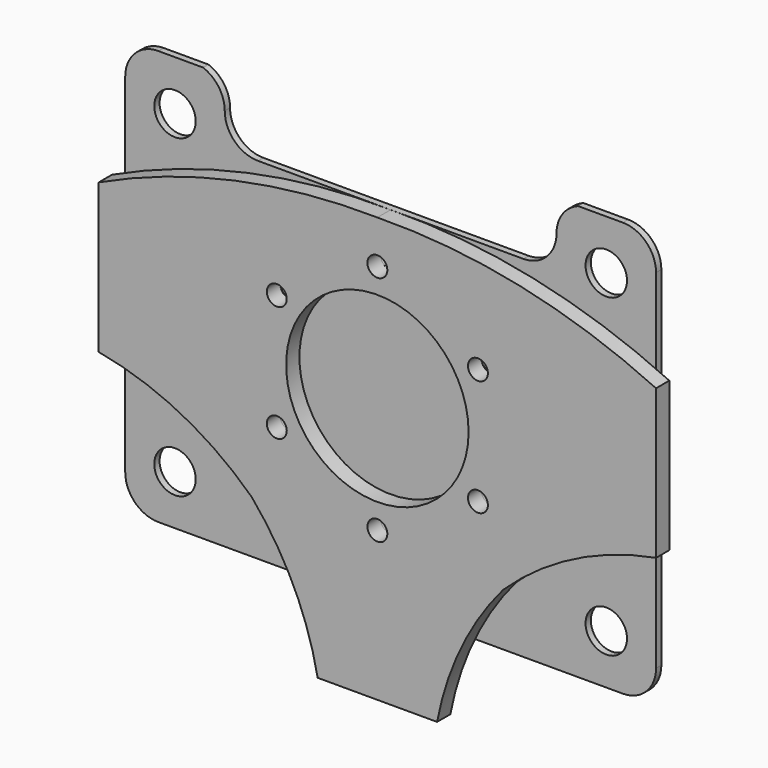
from build123d import *

# Parameters (mm, degrees)
F0_R     = 3
F1_DEPTH = 5
F2_R     = 6.25
F2_R_2   = 3
F3_DEPTH = 2


# Not quite as in the source:
# - a feature names something its author has since deleted; it is built from what else it names


with BuildPart() as f1:
    # F0 (on Front) → F1 (new body)
    with BuildSketch(Plane.XZ):
        with BuildLine():
            ThreePointArc((18, -80), (25.2450835608, -57.9435000854), (37.8911830779, -38.474124356))
            ThreePointArc((37.8911830779, -38.474124356), (59.2223421632, -23.3521866114), (84, -15))
            Line((84, -15), (84, 30))
            ThreePointArc((84, 30), (43.0306603199, 43.8097481595), (0, 48))
            ThreePointArc((0, 48), (-43.0306603199, 43.8097481595), (-84, 30))
            Line((-84, 30), (-84, -15))
            ThreePointArc((-84, -15), (-59.2223421632, -23.3521866114), (-37.8911830779, -38.474124356))
            ThreePointArc((-37.8911830779, -38.474124356), (-25.2450835608, -57.9435000854), (-18, -80))
            Line((-18, -80), (0, -80))
            Line((0, -80), (18, -80))
        make_face()
        with Locations((-30.3108891325, -17.5)):
            Circle(F0_R, mode=Mode.SUBTRACT)
        with Locations((0, -35)):
            Circle(F0_R, mode=Mode.SUBTRACT)
        with Locations((30.3108891325, -17.5)):
            Circle(F0_R, mode=Mode.SUBTRACT)
        with Locations((-30.3108891325, 17.5)):
            Circle(F0_R, mode=Mode.SUBTRACT)
        with BuildLine():
            ThreePointArc((19.2964358267, -19.5933040702), (-25.3663358138, 10.6206877076), (27.5, 0))
            ThreePointArc((27.5, 0), (25.3663358138, -10.6206877076), (19.2964358267, -19.5933040702))
        make_face(mode=Mode.SUBTRACT)
        with Locations((30.3108891325, 17.5)):
            Circle(F0_R, mode=Mode.SUBTRACT)
        with Locations((0, 35)):
            Circle(F0_R, mode=Mode.SUBTRACT)
    extrude(amount=F1_DEPTH)


with BuildPart() as f3:
    # F2 (on Front) → F3 (new body)
    with BuildSketch(Plane.XZ):
        with BuildLine():
            ThreePointArc((-40, 48), (-47.0710678119, 50.9289321881), (-50, 58))
            ThreePointArc((-50, 58), (-51.7877055527, 63.7059810647), (-56.5116439822, 67.3718393228))
            Line((-56.5116439822, 67.3718393228), (-70, 67.3718393228))
            ThreePointArc((-70, 67.3718393228), (-77.0710678119, 64.4429071347), (-80, 57.3718393228))
            Line((-80, 57.3718393228), (-80, -47.6281606772))
            ThreePointArc((-80, -47.6281606772), (-77.0710678119, -54.699228489), (-70, -57.6281606772))
            Line((-70, -57.6281606772), (0, -57.6281606772))
            Line((0, -57.6281606772), (70, -57.6281606772))
            ThreePointArc((70, -57.6281606772), (77.0710678119, -54.699228489), (80, -47.6281606772))
            Line((80, -47.6281606772), (80, 57.3718393228))
            ThreePointArc((80, 57.3718393228), (77.0710678119, 64.4429071347), (70, 67.3718393228))
            Line((70, 67.3718393228), (56.5116439822, 67.3718393228))
            ThreePointArc((56.5116439822, 67.3718393228), (51.7877055527, 63.7059810647), (50, 58))
            ThreePointArc((50, 58), (47.0710678119, 50.9289321881), (40, 48))
            Line((40, 48), (0, 48))
            Line((0, 48), (-40, 48))
        make_face()
        with Locations((-65, -42.6281606772)):
            Circle(F2_R, mode=Mode.SUBTRACT)
        with Locations((-30.3108891325, -17.6374954636)):
            Circle(F2_R_2, mode=Mode.SUBTRACT)
        with Locations((0, -35)):
            Circle(F2_R_2, mode=Mode.SUBTRACT)
        with Locations((65, -42.6281606772)):
            Circle(F2_R, mode=Mode.SUBTRACT)
        with Locations((30.3108891325, -17.6374954636)):
            Circle(F2_R_2, mode=Mode.SUBTRACT)
        with Locations((-30.3108891325, 17.6374954636)):
            Circle(F2_R_2, mode=Mode.SUBTRACT)
        with Locations((-65, 52.3718393228)):
            Circle(F2_R, mode=Mode.SUBTRACT)
        with Locations((30.3108891325, 17.6374954636)):
            Circle(F2_R_2, mode=Mode.SUBTRACT)
        with BuildLine():
            ThreePointArc((0, 32), (-3, 35), (0, 38))
            ThreePointArc((0, 38), (2.1213203436, 37.1213203436), (3, 35))
            ThreePointArc((3, 35), (2.1213203436, 32.8786796564), (0, 32))
        make_face(mode=Mode.SUBTRACT)
        with Locations((65, 52.3718393228)):
            Circle(F2_R, mode=Mode.SUBTRACT)
    extrude(amount=-F3_DEPTH)


solid = Compound([f1.part, f3.part])
